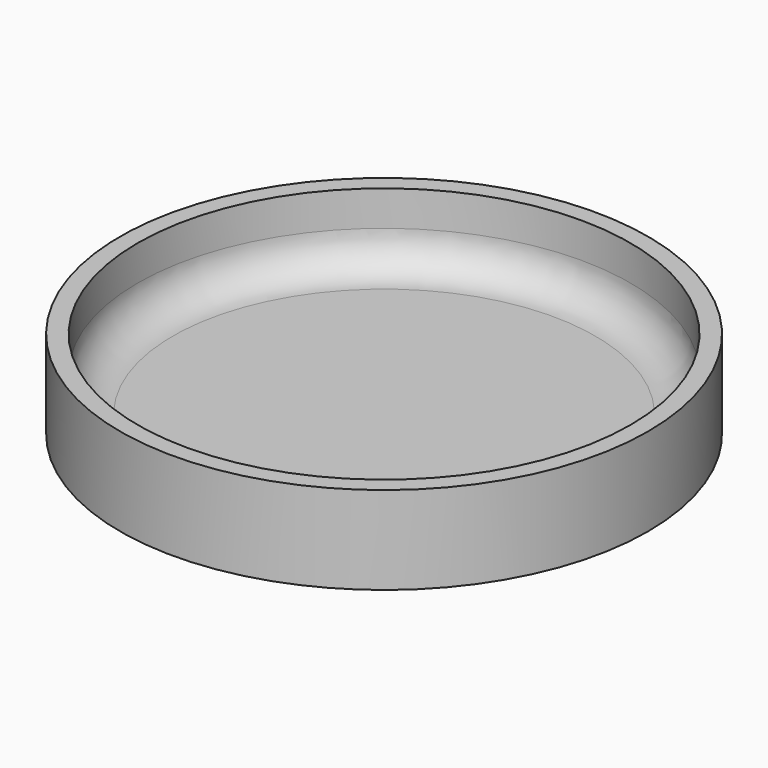
from build123d import *

# Parameters (mm, degrees)
F0_R     = 38.1
F1_DEPTH = 6.35
F2_T     = -2.54
F3_R     = 5.08


with BuildPart() as f1:
    # F0 (on Top) → F1 (new body, symmetric)
    with BuildSketch(Plane.XY):
        Circle(F0_R)
    extrude(amount=F1_DEPTH, both=True)

    # F2
    f2_openings = [f1.faces().sort_by_distance(p)[0] for p in [
        (0, 0, 6.35),
    ]]
    offset(amount=F2_T, openings=f2_openings)

    # F3
    f3_edges = [f1.edges().sort_by_distance(p)[0] for p in [
        (-35.56, 0, -3.81),
    ]]
    fillet(f3_edges, radius=F3_R)


solid = f1.part
